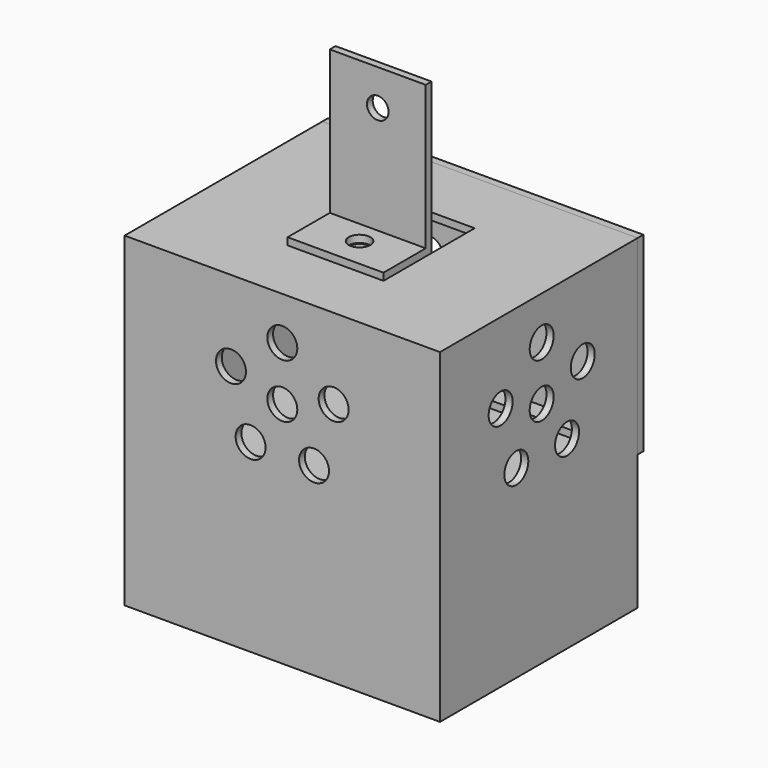
from build123d import *

# Parameters (mm, degrees)
F0_W      = 50.2
F0_H      = 40
F1_DEPTH  = 1.2
F2_DEPTH  = 22.5
F3_W      = 50.2
F3_H      = 40
F4_DEPTH  = 0.6
F5_W      = 25.1
F5_H      = 6
F6_DEPTH  = 0.6
F8_DEPTH  = 30
F9_W      = 50.2
F9_H      = 40
F10_DEPTH = 1.2
F11_W     = 16
F11_H     = 9
F11_R     = 1.5
F12_DEPTH = 1.2
F13_W     = 15
F13_H     = 9
F14_DEPTH = 1.2
F15_R     = 2.5
F16_DEPTH = 1.2
F17_R     = 2.5
F18_DEPTH = 1.2
F19_W     = 16
F19_H     = 10
F19_R     = 1.8
F20_DEPTH = 1.2
F21_W     = 16
F21_H     = 1.2
F22_DEPTH = 24
F23_R     = 1.8
F24_DEPTH = 1.2
F25_W     = 50.2
F25_H     = 30
F25_R     = 2.5
F26_DEPTH = 1.2
F27_W     = 1.2
F27_H     = 1.2
F27_W_2   = 47.4
F27_H_2   = 27.2
F28_DEPTH = 3


with BuildPart() as f1:
    # F0 (on Top) → F1 (new body)
    with BuildSketch(Plane.XY):
        with Locations((25.1, 20)):
            Rectangle(F0_W, F0_H)
    extrude(amount=F1_DEPTH)

    # F0 (on Top) → F2 (join)
    with BuildSketch(Plane.XY):
        Polygon((50.2, 0), (0, 0), (0, 40), (-1.2, 40), (-1.2, -1.2), (51.4, -1.2), (51.4, 40), (50.2, 40), align=None)
    extrude(amount=F2_DEPTH)

    # F3 (on face) → F4 (join)
    with BuildSketch(Plane.XY.offset(22.5)):
        with Locations((25.1, 20)):
            Rectangle(F3_W, F3_H)
        Polygon((50.2, 0), (0, 0), (0, 40), (-1.2, 40), (-1.2, -1.2), (51.4, -1.2), (51.4, 40), (50.2, 40), align=None)
    extrude(amount=F4_DEPTH)

    # F5 (on face) → F6 (cut, through all)
    with BuildSketch(Plane.XY.offset(23.1)):
        with Locations((37.65, 3)):
            Rectangle(F5_W, F5_H)
    extrude(amount=-F6_DEPTH, mode=Mode.SUBTRACT)

    # F7 (on face) → F8 (join)
    with BuildSketch(Plane.XY.offset(23.1)):
        Polygon((-1.2, 40), (-1.2, -1.2), (51.4, -1.2), (51.4, 40), (50.2, 40), (50.2, 6), (50.2, 0), (25.1, 0), (0, 0), (0, 40), align=None)
    extrude(amount=F8_DEPTH)

    # F9 (on face) → F10 (join)
    with BuildSketch(Plane.XY.offset(53.1)):
        with Locations((25.1, 20)):
            Rectangle(F9_W, F9_H)
        Polygon((-1.2, -1.2), (51.4, -1.2), (51.4, 40), (50.2, 40), (50.2, 0), (0, 0), (0, 40), (-1.2, 40), align=None)
    extrude(amount=F10_DEPTH)

    # F11 (on face) → F12 (cut, through all)
    with BuildSketch(Plane.XY.offset(54.3)):
        with Locations((25.1, 24.4)):
            Rectangle(F11_W, F11_H)
        with Locations((25.1, 14.9)):
            Circle(F11_R)
    extrude(amount=-F12_DEPTH, mode=Mode.SUBTRACT)

    # F13 (on face) → F14 (cut, through all)
    with BuildSketch(Plane(origin=(-1.2, 0, 0), x_dir=(0, -1, 0), z_dir=(-1, 0, 0))):
        with Locations((-20, 35.6)):
            Rectangle(F13_W, F13_H)
    extrude(amount=-F14_DEPTH, mode=Mode.SUBTRACT)

    # F15 (on face) → F16 (cut, through all)
    with BuildSketch(Plane.YZ.offset(51.4)):
        with Locations((28.5595086467, 40.8811529494)):
            Circle(F15_R)
        with Locations((20, 47.1)):
            Circle(F15_R)
        with Locations((20, 38.1)):
            Circle(F15_R)
        with Locations((11.4404913533, 40.8811529494)):
            Circle(F15_R)
        with Locations((14.7099327294, 30.8188470506)):
            Circle(F15_R)
        with Locations((25.2900672706, 30.8188470506)):
            Circle(F15_R)
    extrude(amount=-F16_DEPTH, mode=Mode.SUBTRACT)

    # F17 (on face) → F18 (cut, through all)
    with BuildSketch(Plane.XZ.offset(1.2)):
        with Locations((25.1, 47.1)):
            Circle(F17_R)
        with Locations((33.6595086467, 40.8811529494)):
            Circle(F17_R)
        with Locations((30.3900672706, 30.8188470506)):
            Circle(F17_R)
        with Locations((25.1, 38.1)):
            Circle(F17_R)
        with Locations((16.5404913533, 40.8811529494)):
            Circle(F17_R)
        with Locations((19.8099327294, 30.8188470506)):
            Circle(F17_R)
    extrude(amount=-F18_DEPTH, mode=Mode.SUBTRACT)


with BuildPart() as f20:
    # F19 (on face) → F20 (new body)
    with BuildSketch(Plane.XY.offset(54.3)):
        with Locations((25.1, 14.9)):
            Rectangle(F19_W, F19_H)
        with Locations((25.1, 14.9)):
            Circle(F19_R, mode=Mode.SUBTRACT)
    extrude(amount=F20_DEPTH)

    # F21 (on face) → F22 (join)
    with BuildSketch(Plane.XY.offset(55.5)):
        with Locations((25.1, 19.3)):
            Rectangle(F21_W, F21_H)
    extrude(amount=F22_DEPTH)

    # F23 (on face) → F24 (cut, through all)
    with BuildSketch(Plane.XZ.offset(-18.7)):
        with Locations((25.1, 73.5)):
            Circle(F23_R)
    extrude(amount=-F24_DEPTH, mode=Mode.SUBTRACT)


with BuildPart() as f26:
    # F25 (on face) → F26 (new body)
    with BuildSketch(Plane(origin=(0, 40, 0), x_dir=(-1, 0, 0), z_dir=(0, 1, 0))):
        Polygon((1.2, 22.5), (1.2, 54.3), (-51.4, 54.3), (-51.4, 22.5), (-50.2, 22.5), (0, 22.5), align=None)
        with Locations((-25.1, 38.1)):
            Rectangle(F25_W, F25_H, mode=Mode.SUBTRACT)
        with Locations((-25.1, 38.1)):
            Rectangle(F25_W, F25_H)
        with Locations((-30.3900672706, 30.8188470506)):
            Circle(F25_R, mode=Mode.SUBTRACT)
        with Locations((-25.1, 38.1)):
            Circle(F25_R, mode=Mode.SUBTRACT)
        with Locations((-33.6595086467, 40.8811529494)):
            Circle(F25_R, mode=Mode.SUBTRACT)
        with Locations((-25.1, 47.1)):
            Circle(F25_R, mode=Mode.SUBTRACT)
        with Locations((-19.8099327294, 30.8188470506)):
            Circle(F25_R, mode=Mode.SUBTRACT)
        with Locations((-16.5404913533, 40.8811529494)):
            Circle(F25_R, mode=Mode.SUBTRACT)
    extrude(amount=F26_DEPTH)

    # F27 (on face) → F28 (join)
    with BuildSketch(Plane.XZ.offset(-40)):
        with Locations((49.4, 52.3)):
            Rectangle(F27_W, F27_H)
        with Locations((25.1, 52.3)):
            Rectangle(F27_W_2, F27_H)
        with Locations((0.8, 52.3)):
            Rectangle(F27_W, F27_H)
        Polygon((1.4, 52.9), (1.4, 53.1), (0, 53.1), (0, 51.7), (0.2, 51.7), (0.2, 52.9), align=None)
        with Locations((0.8, 38.1)):
            Rectangle(F27_W, F27_H_2)
        with Locations((0.8, 23.9)):
            Rectangle(F27_W, F27_H)
        Polygon((0, 23.1), (1.4, 23.1), (1.4, 23.3), (0.2, 23.3), (0.2, 24.5), (0, 24.5), align=None)
        with Locations((25.1, 23.9)):
            Rectangle(F27_W_2, F27_H)
        with Locations((49.4, 23.9)):
            Rectangle(F27_W, F27_H)
        Polygon((50.2, 23.1), (50.2, 24.5), (50, 24.5), (50, 23.3), (48.8, 23.3), (48.8, 23.1), align=None)
        with Locations((49.4, 38.1)):
            Rectangle(F27_W, F27_H_2)
        Polygon((50.2, 51.7), (50.2, 53.1), (48.8, 53.1), (48.8, 52.9), (50, 52.9), (50, 51.7), align=None)
    extrude(amount=F28_DEPTH)


solid = Compound([f1.part, f20.part, f26.part])
